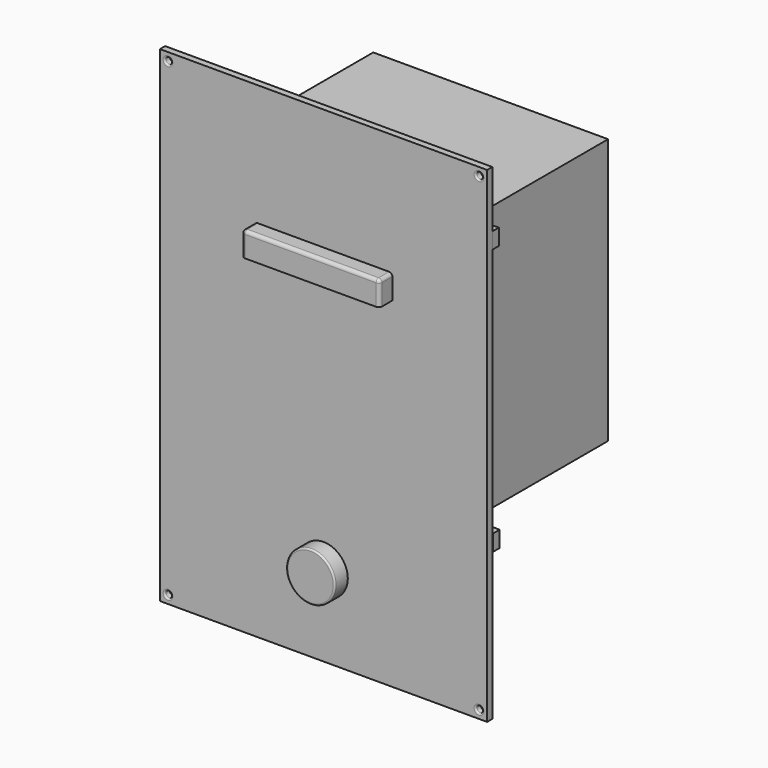
from build123d import *

# Parameters (mm, degrees)
F0_W      = 202
F0_H      = 300
F1_DEPTH  = 4
F2_R      = 2
F3_DEPTH  = 5
F4_R      = 15
F5_DEPTH  = 10
F6_R      = 1
F7_W      = 85
F7_H      = 15
F8_DEPTH  = 10
F9_R      = 2
F10_T     = 2
F11_W     = 81
F11_H     = 13
F12_DEPTH = 10
F2_W      = 82
F2_H      = 5
F13_DEPTH = 25
F14_R     = 1
F15_W     = 202
F15_H     = 10
F16_DEPTH = 5
F17_W     = 145
F17_H     = 164
F17_W_2   = 90
F17_H_2   = 18
F18_DEPTH = 120


# Not quite as in the source:
# - a shell that OpenCascade refuses in one call is made with other operations: the cavity is built on its own and cut out
# - a feature names something its author has since deleted; it is built from what else it names


with BuildPart() as f1:
    # F0 (on Front) → F1 (new body)
    with BuildSketch(Plane.XZ):
        with Locations((-42.2897736542, 111.9996137917)):
            Rectangle(F0_W, F0_H)
    extrude(amount=F1_DEPTH)

    # F2 (on face) → F3 (cut)
    with BuildSketch(Plane.XZ.offset(4)):
        with Locations((-138.2897736542, -33.0003862083)):
            Circle(F2_R)
        with Locations((-138.2897736542, 256.9996137917)):
            Circle(F2_R)
        with Locations((53.7102263458, 256.9996137917)):
            Circle(F2_R)
        with Locations((53.7102263458, -33.0003862083)):
            Circle(F2_R)
    extrude(amount=-F3_DEPTH, mode=Mode.SUBTRACT)

    # F2 (on face) → F13 (cut)
    with BuildSketch(Plane.XZ.offset(4)):
        with Locations((-42.2897736542, 179.4996137917)):
            Rectangle(F2_W, F2_H)
    extrude(amount=-F13_DEPTH, mode=Mode.SUBTRACT)

    # F14
    f14_edges = [f1.edges().sort_by_distance(p)[0] for p in [
        (-140.289774, -4, 256.999614),
        (-140.289774, -4, -33.000386),
        (51.710226, -4, -33.000386),
        (51.710226, -4, 256.999614),
    ]]
    fillet(f14_edges, radius=F14_R)


with BuildPart() as f5:
    # F4 (on face) → F5 (new body)
    with BuildSketch(Plane.XZ.offset(4)):
        with Locations((-42.2897736542, 11.9996137917)):
            Circle(F4_R)
    extrude(amount=F5_DEPTH)

    # F6
    f6_edges = [f5.edges().sort_by_distance(p)[0] for p in [
        (-57.289774, -14, 11.999614),
    ]]
    fillet(f6_edges, radius=F6_R)


with BuildPart() as f8:
    # F7 (on face) → F8 (new body)
    with BuildSketch(Plane.XZ.offset(4)):
        with Locations((-42.2897736542, 179.4996137917)):
            Rectangle(F7_W, F7_H)
    extrude(amount=F8_DEPTH)

    # F9
    f9_edges = [f8.edges().sort_by_distance(p)[0] for p in [
        (-84.789774, -14, 179.499614),
        (-42.289774, -14, 186.999614),
        (0.210226, -14, 179.499614),
        (0.210226, -9, 186.999614),
        (-84.789774, -9, 186.999614),
    ]]
    fillet(f9_edges, radius=F9_R)

    # F10: shell of thickness 2, made by hand


with BuildPart() as f10_core1:
    # F10_t2: copy of F8
    add(f8.part)

    # the walls: a layer under each face that stays
    f10_faces = [f10_core1.faces().sort_by_distance(p)[0] for p in [
        (-42.2897736542, -8, 186.9996137917),
        (-42.2897736542, -4, 179.4996137917),
        (0.2102263458, -8, 178.4996137917),
        (-84.7897736542, -8, 178.4996137917),
        (-42.2897736542, -14, 178.4996137917),
    ]]
    thicken(f10_faces, amount=-F10_T, mode=Mode.SUBTRACT)


with BuildPart() as f8_1:
    add(f8.part)

    # what is left inside the walls is the cavity
    f10_cavity = [f10_core1.part.solids().sort_by_distance(p)[0] for p in [
        (-42.289774, -6.02, 176.332947),
    ]]
    add(f10_cavity, mode=Mode.SUBTRACT)

    # F11 (on face) → F12 (cut)
    with BuildSketch(Plane.XZ.offset(6)):
        with Locations((-42.2897736542, 178.4996137917)):
            Rectangle(F11_W, F11_H)
    extrude(amount=-F12_DEPTH, mode=Mode.SUBTRACT)


with BuildPart() as f16:
    # F15 (on face) → F16 (new body)
    with BuildSketch(Plane.XZ):
        with Locations((-42.2897736542, 221.9996137917)):
            Rectangle(F15_W, F15_H)
    extrude(amount=-F16_DEPTH)


with BuildPart() as f16b:
    # F15 (on face) → F16, piece 2 (new body)
    with BuildSketch(Plane.XZ):
        with Locations((-41.7558064461, 57.9996137917)):
            Rectangle(F15_W, F15_H)
    extrude(amount=-F16_DEPTH)


with BuildPart() as f18:
    # F17 (on face) → F18 (new body)
    with BuildSketch(Plane(origin=(0, 5, 0), x_dir=(-1, 0, 0), z_dir=(0, 1, 0))):
        with Locations((42.2897736542, 134.9996137917)):
            Rectangle(F17_W, F17_H)
        with Locations((42.2897736542, 177.9996137917)):
            Rectangle(F17_W_2, F17_H_2, mode=Mode.SUBTRACT)
    extrude(amount=F18_DEPTH)


solid = Compound([f1.part, f5.part, f8_1.part, f16.part, f16b.part, f18.part])
